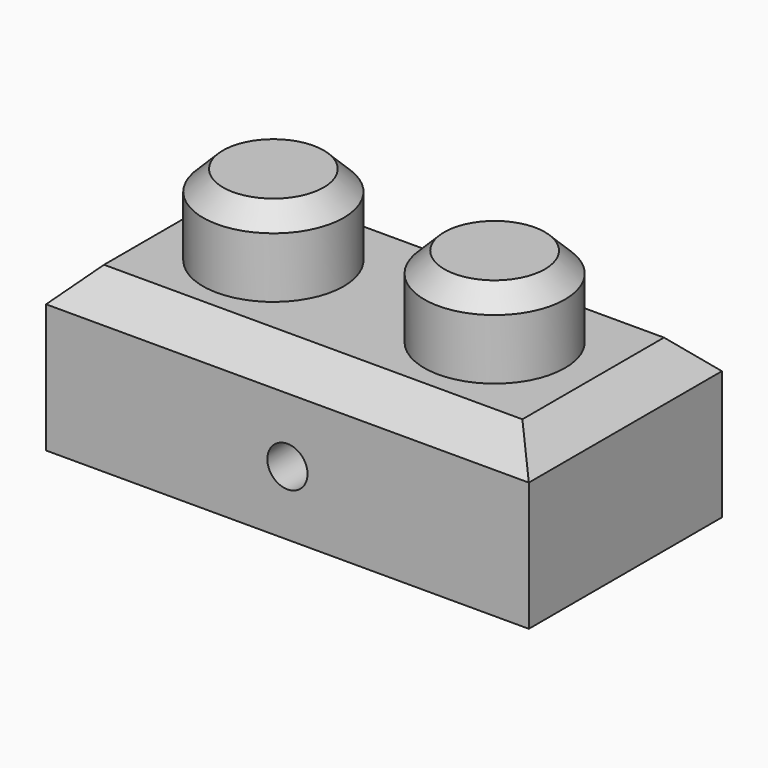
from build123d import *

# Parameters (mm, degrees)
F0_W      = 76.2
F0_H      = 38.1
F1_DEPTH  = 25.4
F2_SIZE   = 5.08
F3_R      = 11.1125
F4_DEPTH  = 12.7
F5_SIZE   = 3.175
F7_T      = 7.9375
F6_R      = 3.175
F8_DEPTH  = 7.9375
F9_R      = 3.175
F10_DEPTH = 7.9375


# Not quite as in the source:
# - a shell that OpenCascade refuses in one call is made with other operations: the cavity is built on its own and cut out


with BuildPart() as f1:
    # F0 (on Top) → F1 (new body)
    with BuildSketch(Plane.XY):
        with Locations((-12.72226125, 10.7161214997)):
            Rectangle(F0_W, F0_H)
    extrude(amount=F1_DEPTH)

    # F2
    f2_edges = [f1.edges().sort_by_distance(p)[0] for p in [
        (-50.822261, 10.716121, 25.4),
        (-12.722261, 29.766121, 25.4),
        (-12.722261, -8.333879, 25.4),
        (25.377739, 10.716121, 25.4),
    ]]
    chamfer(f2_edges, length=F2_SIZE)

    # F3 (on face) → F4 (join)
    with BuildSketch(Plane.XY.offset(25.4)):
        with Locations((-30.18476125, 10.7161214997)):
            Circle(F3_R)
        with Locations((4.74023875, 10.7161214997)):
            Circle(F3_R)
    extrude(amount=F4_DEPTH)

    # F5
    f5_edges = [f1.edges().sort_by_distance(p)[0] for p in [
        (-41.297261, 10.716121, 38.1),
        (-6.372261, 10.716121, 38.1),
    ]]
    chamfer(f5_edges, length=F5_SIZE)

    # F7: shell of thickness 7.9375, made by hand


with BuildPart() as f7_core1:
    # F7_t2: copy of F1
    add(f1.part)

    # the walls: a layer under each face that stays
    f7_faces = [f7_core1.faces().sort_by_distance(p)[0] for p in [
        (-41.29726125, 10.7161214997, 30.1625),
        (-39.70976125, 10.7161214997, 36.5125),
        (-12.72226125, 10.7161214997, 25.4),
        (-30.18476125, 10.7161214997, 38.1),
        (-48.28226125, 10.7161214997, 22.86),
        (-12.72226125, 27.2261214997, 22.86),
        (-12.72226125, -5.7938785003, 22.86),
        (22.83773875, 10.7161214997, 22.86),
        (-6.37226125, 10.7161214997, 30.1625),
        (-50.82226125, 10.7161214997, 10.16),
        (-12.72226125, 29.7661214997, 10.16),
        (-12.72226125, -8.3338785003, 10.16),
        (25.37773875, 10.7161214997, 10.16),
        (-4.78476125, 10.7161214997, 36.5125),
        (4.74023875, 10.7161214997, 38.1),
    ]]
    thicken(f7_faces, amount=-F7_T, mode=Mode.SUBTRACT)

    # F7_s3 → F7_t4 (revolve, cut)
    with BuildSketch(Plane.XZ.offset(-10.7161214997)):
        Polygon((-18.99288625, 25.479375), (-27.00976125, 25.4), (-27.00976125, 17.4625), (-19.07226125, 17.4625), align=None)
    revolve(axis=Axis((-30.18476125, 10.7161214997, 25.4), (0, 0, 1)), mode=Mode.SUBTRACT)

    # F7_s5 → F7_t6 (revolve, cut)
    with BuildSketch(Plane.XZ.offset(-10.7161214997)):
        Polygon((15.93211375, 25.479375), (15.85273875, 17.4625), (7.91523875, 17.4625), (7.91523875, 25.4), align=None)
    revolve(axis=Axis((4.74023875, 10.7161214997, 25.4), (0, 0, 1)), mode=Mode.SUBTRACT)


with BuildPart() as f1_1:
    add(f1.part)

    # what is left inside the walls is the cavity
    f7_cavity = [f7_core1.part.solids().sort_by_distance(p)[0] for p in [
        (-12.722261, 7.011955, 0.079375),
    ]]
    add(f7_cavity, mode=Mode.SUBTRACT)

    # F6 (on face) → F8 (cut)
    with BuildSketch(Plane.XZ.offset(8.3338785003)):
        with Locations((-12.72226125, 10.16)):
            Circle(F6_R)
    extrude(amount=-F8_DEPTH, mode=Mode.SUBTRACT)

    # F9 (on face) → F10 (cut)
    with BuildSketch(Plane(origin=(0, 29.7661214997, 0), x_dir=(-1, 0, 0), z_dir=(0, 1, 0))):
        with Locations((12.72226125, 10.16)):
            Circle(F9_R)
    extrude(amount=-F10_DEPTH, mode=Mode.SUBTRACT)


solid = f1_1.part
